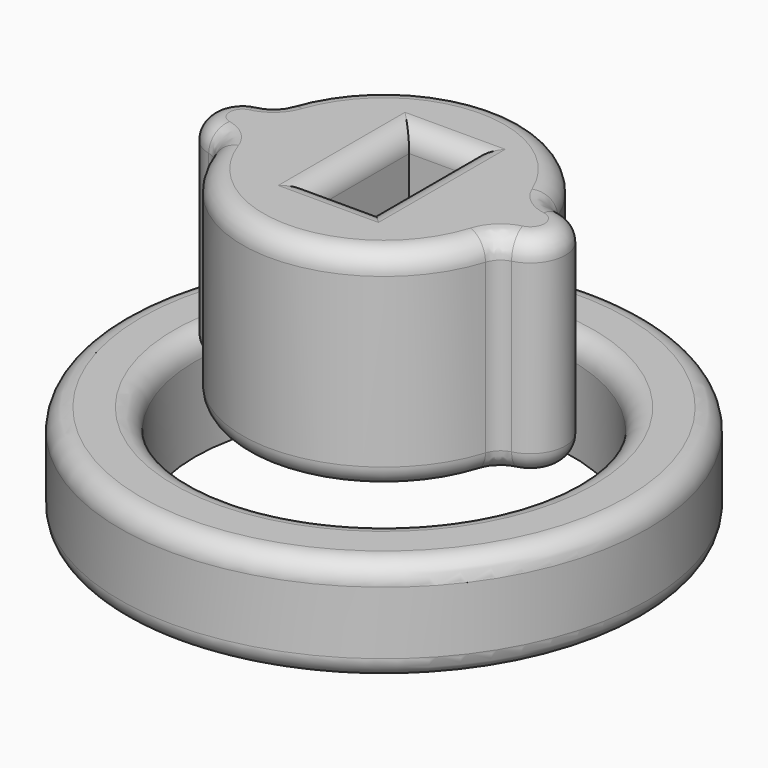
from build123d import *

# Parameters (mm, degrees)
F0_R     = 63.9179565319
F0_R_2   = 45.7330498598
F1_DEPTH = 25.4
F0_W     = 14.1024817713
F0_H     = 28.2049654052
F2_DEPTH = 25.4
F3_DEPTH = 25.4
F4_F1_R  = 5.08
F4_F2_R  = 5.08
F4_F3_R  = 5.08
F5_R     = 5.08


# Not quite as in the source:
# - a feature of the source that left no trace in its solid (it failed there, or was rolled back) is left out


with BuildPart() as f1:
    # F0 (on Top) → F1 (new body)
    with BuildSketch(Plane.XY):
        Circle(F0_R)
        Circle(F0_R_2, mode=Mode.SUBTRACT)
    extrude(amount=-F1_DEPTH)

    # F5
    f5_edges = [f1.edges().sort_by_distance(p)[0] for p in [
        (63.917957, 0, -12.7),
        (-63.917957, 0, 0),
        (-63.917957, 0, -25.4),
        (-45.73305, 0, 0),
    ]]
    fillet(f5_edges, radius=F5_R)


with BuildPart() as f2:
    # F0 (on Top) → F2 (new body)
    with BuildSketch(Plane.XY):
        with BuildLine():
            ThreePointArc((-33.2797462544, 8.1357294422), (-42.4543094539, 0), (-33.2797462544, -8.1357294422))
            ThreePointArc((-33.2797462544, -8.1357294422), (0.5813538288, -34.2548337033), (33.5366512199, -7.0017590123))
            ThreePointArc((33.5366512199, -7.0017590123), (42.7369569293, 1.8575969402), (32.8026434596, 9.8852509515))
            ThreePointArc((32.8026434596, 9.8852509515), (-0.9067045534, 34.2477662216), (-33.2797462544, 8.1357294422))
        make_face()
        with Locations((0.7195149083, 1.4390288852)):
            Rectangle(F0_W, F0_H, mode=Mode.SUBTRACT)
    extrude(amount=F2_DEPTH)

    # F3 (add): a face of the model
    f3_faces = [f2.faces().sort_by_distance(p)[0] for p in [
        (0.5628010063, -33.1616546129, 25.4),
    ]]
    extrude(f3_faces, amount=F3_DEPTH)

    # F4: fillet of radius 5.08 on 15 edges, made by hand

    # F4_f1
    f4_f1_edges = [f2.edges().sort_by_distance(p)[0] for p in [
        (-33.2797462544, -8.1357294422, 25.4),
        (33.5366512199, -7.0017590123, 25.4),
        (32.8026434596, 9.8852509515, 25.4),
        (-33.2797462544, 8.1357294422, 25.4),
    ]]
    fillet(f4_f1_edges, radius=F4_F1_R)

    # F4_f2
    f4_f2_edges = [f2.edges().sort_by_distance(p)[0] for p in [
        (-6.3317259774, 1.4390288852, 50.8),
        (0.7195149083, 15.5415115878, 50.8),
        (7.7707557939, 1.4390288852, 50.8),
        (0.7195149083, -12.6634538174, 50.8),
    ]]
    fillet(f4_f2_edges, radius=F4_F2_R)

    # F4_f3
    f4_f3_edges = [f2.edges().sort_by_distance(p)[0] for p in [
        (0.5788820282, -34.2548755641, 50.8),
        (0.5788820282, -34.2548755641, 0),
        (42.7369569293, 1.8575969402, 50.8),
        (42.7369569293, 1.8575969402, 0),
        (-0.9091758401, 34.2477007054, 50.8),
        (-42.4543094539, 0, 50.8),
        (-42.4543094539, 0, 0),
        (-33.7678946689, 9.162035776, 0),
        (-33.7678946689, -9.162035776, 0),
        (-33.7678946689, 9.162035776, 50.8),
        (-33.7678946689, -9.162035776, 50.8),
        (33.2444872281, 10.932568882, 50.8),
        (34.0677019889, -8.0067892826, 0),
        (33.2444872281, 10.932568882, 0),
        (34.0677019889, -8.0067892826, 50.8),
    ]]
    fillet(f4_f3_edges, radius=F4_F3_R)


solid = Compound([f1.part, f2.part])
